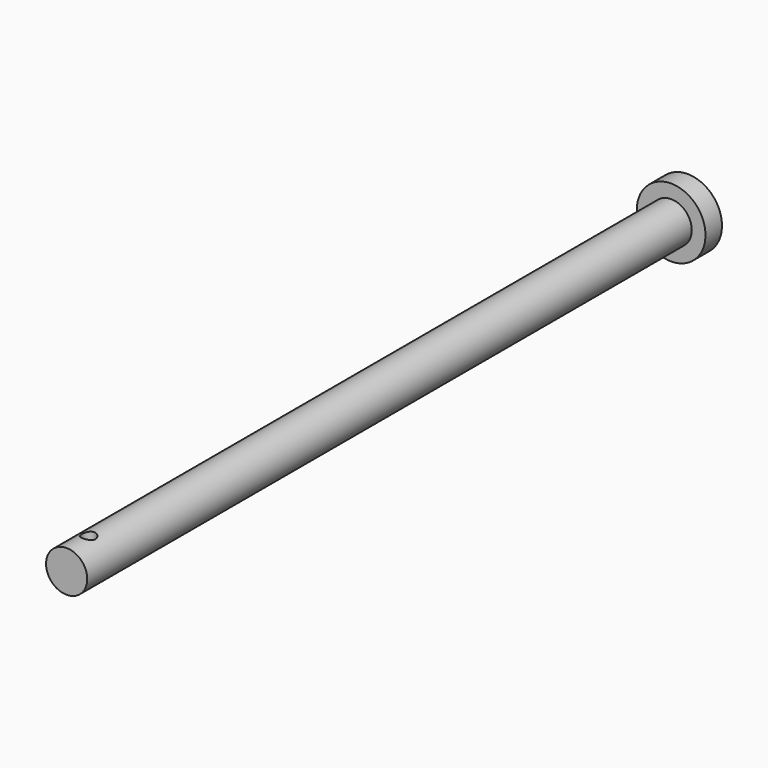
from build123d import *

# Parameters (mm, degrees)
F0_R     = 1.5
F1_DEPTH = 55
F2_R     = 2.5
F2_R_2   = 1.5
F3_DEPTH = 1.5
F4_R     = 0.5
F5_DEPTH = 2.5


with BuildPart() as f1:
    # F0 (on Front) → F1 (new body)
    with BuildSketch(Plane.XZ):
        Circle(F0_R)
    extrude(amount=F1_DEPTH)

    # F2 (on face) → F3 (join)
    with BuildSketch(Plane(origin=(0, 0, 0), x_dir=(-1, 0, 0), z_dir=(0, 1, 0))):
        Circle(F2_R)
        Circle(F2_R_2, mode=Mode.SUBTRACT)
        Circle(F2_R_2)
    extrude(amount=F3_DEPTH)

    # F4 (on Top) → F5 (cut, symmetric)
    with BuildSketch(Plane.XY):
        with Locations((0, -53)):
            Circle(F4_R)
    extrude(amount=F5_DEPTH, both=True, mode=Mode.SUBTRACT)


solid = f1.part
